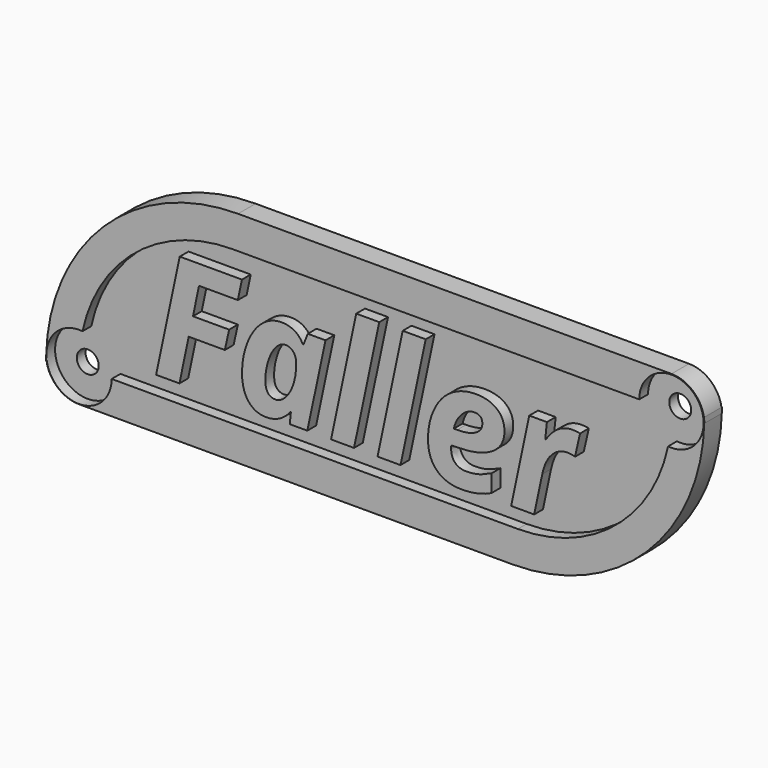
from build123d import *

# Parameters (mm, degrees)
F0_R         = 2
F1_DEPTH     = 4
F2_R         = 5.9562194164
F2_R_2       = 5.8683350072
F3_DEPTH     = 2
F5_DEPTH     = 2
F6_TEXT_SIZE = 28.535424997
F7_DEPTH     = 2


# Not quite as in the source:
# - Text() gives the source's letters only with a copy of the font that has no kerning and outlines rounded to 1/6400 em; it was checked with that copy


with BuildPart() as f1:
    # F0 (on Front) → F1 (new body)
    with BuildSketch(Plane.XZ):
        with BuildLine():
            ThreePointArc((0.0071463796, 5.707245009), (1.8621581679, 1.6550874609), (6, 0))
            Line((6, 0), (85, 0))
            ThreePointArc((85, 0), (109.4974123601, 10.0024643683), (119.9928536204, 34.292754991))
            ThreePointArc((119.9928536204, 34.292754991), (118.1378418321, 38.3449125391), (114, 40))
            Line((114, 40), (35, 40))
            ThreePointArc((35, 40), (10.5025876399, 29.9975356317), (0.0071463796, 5.707245009))
        make_face()
        with Locations((6, 6)):
            Circle(F0_R, mode=Mode.SUBTRACT)
        with Locations((114, 34)):
            Circle(F0_R, mode=Mode.SUBTRACT)
    extrude(amount=F1_DEPTH)

    # F2 (on face) → F3 (cut)
    with BuildSketch(Plane.XZ.offset(4)):
        with Locations((6, 6)):
            Circle(F2_R)
        with Locations((114, 34)):
            Circle(F2_R_2)
    extrude(amount=-F3_DEPTH, mode=Mode.SUBTRACT)

    # F4 (on face) → F5 (cut)
    with BuildSketch(Plane.XZ.offset(4)):
        with BuildLine():
            ThreePointArc((6.6335098167, 11.9224332033), (10.4300041313, 9.9814084358), (11.9562194164, 6))
            Line((11.9562194164, 6), (86, 6))
            ThreePointArc((86, 6), (103.6152107214, 12.2352498007), (113.3850472186, 28.1639749115))
            ThreePointArc((113.3850472186, 28.1639749115), (109.6384575726, 30.0738946256), (108.1316649928, 34))
            Line((108.1316649928, 34), (34, 34))
            ThreePointArc((34, 34), (16.4191599986, 27.7925231409), (6.6335098167, 11.9224332033))
        make_face()
    extrude(amount=-F5_DEPTH, mode=Mode.SUBTRACT)

    # F6 (on face) → F7 (join)
    with BuildSketch(Plane.XZ.offset(2)):
        with Locations((19.3224102453, 9.2991655032)):
            Text('Faller', F6_TEXT_SIZE, font='Open Sans', font_style=FontStyle.BOLDITALIC, text_align=(TextAlign.LEFT, TextAlign.BOTTOM))
    extrude(amount=F7_DEPTH)


with BuildPart() as f1b:
    # F0 (on Front) → F1, piece 2 (new body)
    with BuildSketch(Plane.XZ):
        with BuildLine():
            ThreePointArc((0, 5), (0.0017866405, 5.3536405568), (0.0071463796, 5.707245009))
            ThreePointArc((0.0071463796, 5.707245009), (0.001786861, 5.8535788988), (0, 6))
            Line((0, 6), (0, 5))
        make_face()
    extrude(amount=F1_DEPTH)


with BuildPart() as f1c:
    # F0 (on Front) → F1, piece 3 (new body)
    with BuildSketch(Plane.XZ):
        with BuildLine():
            ThreePointArc((120, 35), (119.9982133595, 34.6463594432), (119.9928536204, 34.292754991))
            ThreePointArc((119.9928536204, 34.292754991), (119.998213139, 34.1464211012), (120, 34))
            Line((120, 34), (120, 35))
        make_face()
    extrude(amount=F1_DEPTH)


solid = Compound([f1.part, f1b.part, f1c.part])
